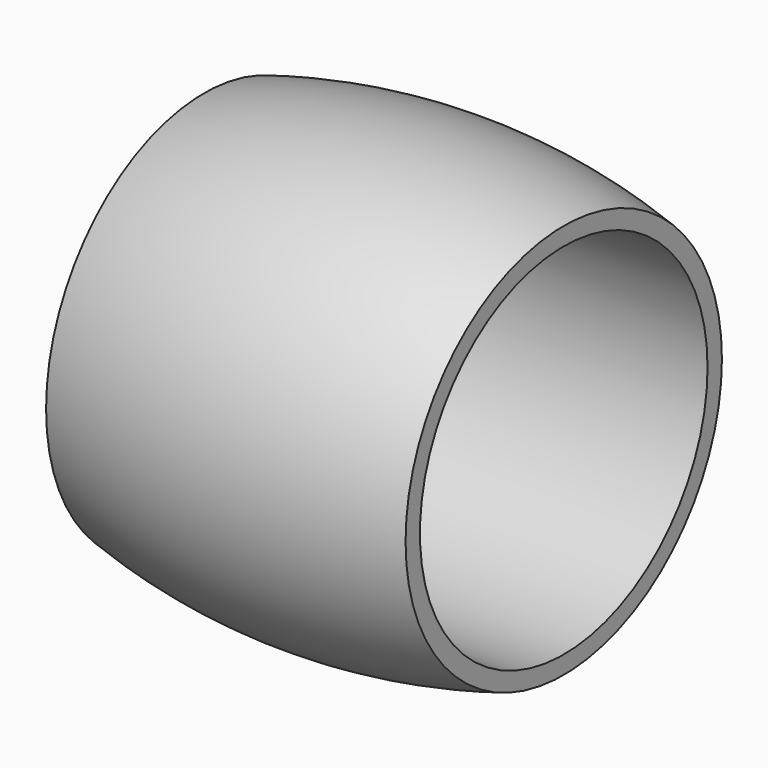
from build123d import *

# Parameters (mm, degrees)
F13_W          = 12.7856880426
F13_H          = 2.7000820846
F14_DEPTH      = 0.635
F14_DEPTH_BACK = 0.635


# Not quite as in the source:
# - a feature of the source that left no trace in its solid (it failed there, or was rolled back) is left out
# - the program builds the solid bodies; features that only make, move or delete a surface that nothing else refers to are left out


with BuildPart() as f3:
    # F2 (on plane+point) → F3 (revolve)
    with BuildSketch(Plane.XY):
        with BuildLine():
            Line((-25.4, -44.7680812202), (-25.4, -47.3080812202))
            Line((-25.4, -47.3080812202), (25.4, -47.3080812202))
            Line((25.4, -47.3080812202), (25.4, -44.7680812202))
            ThreePointArc((25.4, -44.7680812202), (0, -41.2899077912), (-25.4, -44.7680812202))
        make_face()
    revolve(axis=Axis((0, -72.7080783897, 0), (1, 0, 0)))


with BuildPart() as f14:
    # F13 (on line) → F14 (new body, two sides)
    with BuildSketch(Plane.YZ.offset(-31.1320461684)) as f14_sk:
        with BuildLine():
            Line((-79.4192776084, 3.1777741387), (-87.9828110337, -0.2195611014))
            Line((-87.9828110337, -0.2195611014), (-79.3269872665, -4.8583555035))
            Line((-79.3269872665, -4.8583555035), (-58.7705560029, -4.8583555035))
            ThreePointArc((-58.7705560029, -4.8583555035), (-62.1628887785, -0.8402906824), (-58.7705560029, 3.1777741387))
            Line((-58.7705560029, 3.1777741387), (-79.4192776084, 3.1777741387))
        make_face()
        with Locations((-72.628326714, -0.4799846502)):
            Rectangle(F13_W, F13_H, mode=Mode.SUBTRACT)
    extrude(amount=F14_DEPTH)
    extrude(f14_sk.sketch, amount=-F14_DEPTH_BACK)


solid = Compound([f3.part, f14.part])
